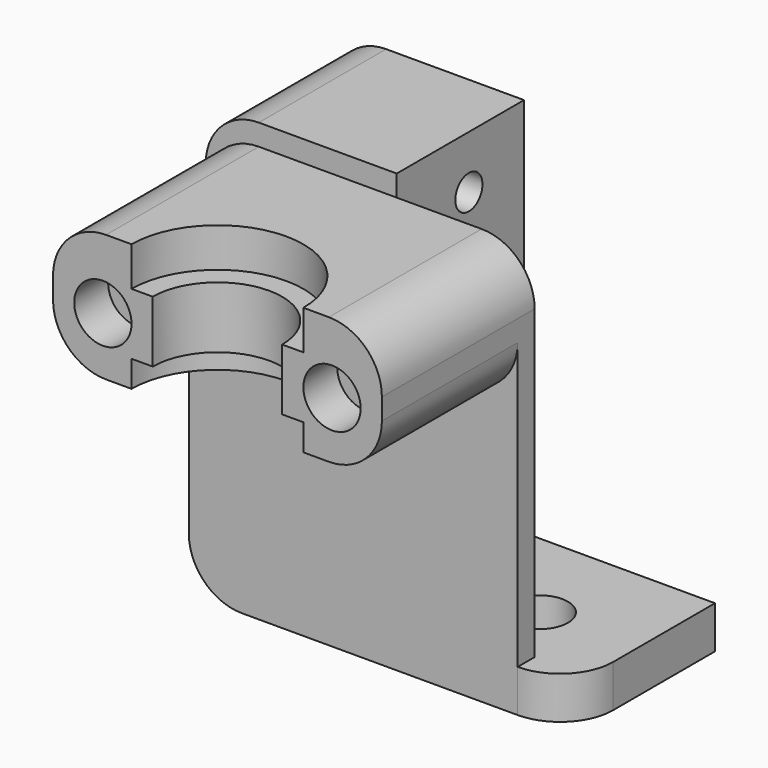
from build123d import *

# Parameters (mm, degrees)
F1_DEPTH     = 15
F2_R         = 1.6
F3_DEPTH     = 36.001
F4_R         = 2.7
F5_DEPTH     = 25
F8_DEPTH     = 3.7
F10_DEPTH    = 5.8
F12_DEPTH    = 2.5
F13_R        = 2.7
F14_DEPTH    = 4
F15_R        = 3.25
F16_DEPTH    = 3.5
F17_W        = 31
F17_H        = 2
F18_DEPTH    = 25.9
F19_W        = 5
F19_H        = 4
F20_DEPTH    = 2
F21_R        = 5
F22_T1_DEPTH = 40


# Not quite as in the source:
# - a fillet or chamfer that OpenCascade refuses, or shapes differently, is made with other operations: its cross-section is extruded or revolved along the edge and cut away or added


with BuildPart() as f1:
    # F0 (on Front) → F1 (new body)
    with BuildSketch(Plane.XZ):
        Polygon((0, 0), (0, 35.9), (-18, 35.9), (-18, -4), (18, -4), (18, 0), align=None)
    extrude(amount=F1_DEPTH)

    # F2 (on face) → F3 (cut, through all)
    with BuildSketch(Plane(origin=(-18, 0, 0), x_dir=(0, -1, 0), z_dir=(-1, 0, 0))):
        with Locations((6.5, 30.9)):
            Circle(F2_R)
    extrude(amount=-F3_DEPTH, mode=Mode.SUBTRACT)

    # F4 (on face) → F5 (cut)
    with BuildSketch(Plane.XY):
        with Locations((8.8, -9.2)):
            Circle(F4_R)
    extrude(amount=-F5_DEPTH, mode=Mode.SUBTRACT)

    # F7 (on offset) → F8 (join)
    with BuildSketch(Plane.XY.offset(33.9)):
        with BuildLine():
            Line((13, -15), (-18, -15))
            Line((-18, -15), (-18, -33))
            Line((-18, -33), (-10.6, -33))
            ThreePointArc((-10.6, -33), (-2.5, -24.9), (5.6, -33))
            Line((5.6, -33), (13, -33))
            Line((13, -33), (13, -15))
        make_face()
    extrude(amount=-F8_DEPTH)

    # F9 (on face) → F10 (join)
    with BuildSketch(Plane(origin=(0, 0, 30.2), x_dir=(1, 0, 0), z_dir=(0, 0, -1))):
        with BuildLine():
            Line((0, 15), (13, 15))
            Line((13, 15), (13, 33))
            Line((13, 33), (5.6, 33))
            Line((5.6, 33), (3.6, 33))
            ThreePointArc((3.6, 33), (-2.5, 26.9), (-8.6, 33))
            Line((-8.6, 33), (-10.6, 33))
            Line((-10.6, 33), (-18, 33))
            Line((-18, 33), (-18, 15))
            Line((-18, 15), (0, 15))
        make_face()
    extrude(amount=F10_DEPTH)

    # F11 (on face) → F12 (join)
    with BuildSketch(Plane(origin=(0, 0, 24.4), x_dir=(1, 0, 0), z_dir=(0, 0, -1))):
        with BuildLine():
            Line((13, 15), (13, 33))
            Line((13, 33), (5.6, 33))
            ThreePointArc((5.6, 33), (-2.5, 24.9), (-10.6, 33))
            Line((-10.6, 33), (-18, 33))
            Line((-18, 33), (-18, 15))
            Line((-18, 15), (13, 15))
        make_face()
    extrude(amount=F12_DEPTH)

    # F13 (on face) → F14 (cut)
    with BuildSketch(Plane.XZ.offset(33)):
        with Locations((-13.3, 27.3)):
            Circle(F13_R)
        with Locations((8.3, 27.3)):
            Circle(F13_R)
    extrude(amount=-F14_DEPTH, mode=Mode.SUBTRACT)

    # F15 (on face) → F16 (cut)
    with BuildSketch(Plane(origin=(-18, 0, 0), x_dir=(0, -1, 0), z_dir=(-1, 0, 0))):
        with Locations((6.5, 30.9)):
            Circle(F15_R)
    extrude(amount=-F16_DEPTH, mode=Mode.SUBTRACT)

    # F17 (on face) → F18 (join, through all)
    with BuildSketch(Plane(origin=(0, 0, 21.9), x_dir=(1, 0, 0), z_dir=(0, 0, -1))):
        with Locations((-2.5, 16)):
            Rectangle(F17_W, F17_H)
    extrude(amount=F18_DEPTH)

    # F19 (on face) → F20 (join, through all)
    with BuildSketch(Plane.XZ.offset(15)):
        with Locations((15.5, -2)):
            Rectangle(F19_W, F19_H)
    extrude(amount=F20_DEPTH)

    # F21
    f21_edges = [f1.edges().sort_by_distance(p)[0] for p in [
        (-18, -25, 21.9),
        (13, -24, 33.9),
        (13, -25, 21.9),
        (-18, -8.5, -4),
        (18, -17, -2),
        (-18, -24, 33.9),
    ]]
    fillet(f21_edges, radius=F21_R)

    # F22: fillet of radius 5 on 1 edges, made by hand

    # F22_s2 → F22_t1 (cut)
    with BuildSketch(Plane.XZ.offset(-12.5)):
        with BuildLine():
            ThreePointArc((-18, 30.9), (-16.535534, 34.435534), (-13, 35.9))
            Line((-13, 35.9), (-18, 35.9))
            Line((-18, 35.9), (-18, 30.9))
        make_face()
    extrude(amount=F22_T1_DEPTH, mode=Mode.SUBTRACT)


solid = f1.part
